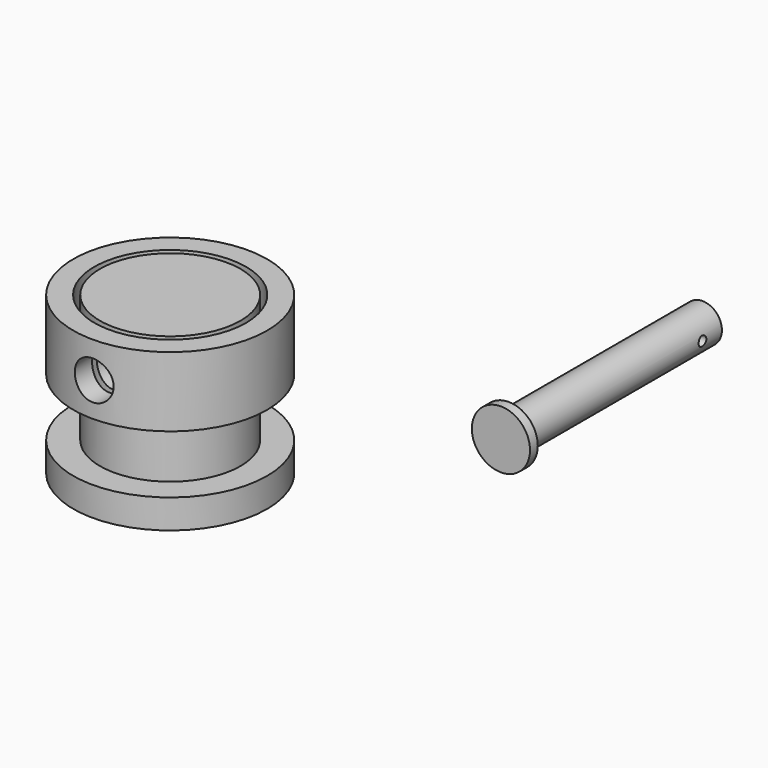
from build123d import *

# Parameters (mm, degrees)
F0_R          = 10
F0_R_2        = 7.83
F1_DEPTH      = 7
F1_DEPTH_BACK = 0.2
F3_R          = 7.25
F4_DEPTH      = 7.2
F4_DEPTH_BACK = 6
F5_START      = 6
F3_R_2        = 10
F3_R_3        = 7.83
F5_DEPTH      = 3
F2_R          = 2
F10_DEPTH     = 93.8892550597
F7_R          = 2
F11_DEPTH     = 25
F7_R_2        = 3
F12_DEPTH     = 1
F13_R         = 0.5
F14_DEPTH     = 25


# Not quite as in the source:
# - a feature of the source that left no trace in its solid (it failed there, or was rolled back) is left out


with BuildPart() as f1:
    # F0 (on Top) → F1 (new body, two sides)
    with BuildSketch(Plane.XY) as f1_sk:
        with Locations((-31.695947051, 83.8882550597)):
            Circle(F0_R)
        with Locations((-31.695947051, 83.8882550597)):
            Circle(F0_R_2, mode=Mode.SUBTRACT)
    extrude(amount=F1_DEPTH)
    extrude(f1_sk.sketch, amount=-F1_DEPTH_BACK)


with BuildPart() as f4:
    # F3 (on face) → F4 (new body, two sides)
    with BuildSketch(Plane(origin=(0, 0, -0.2), x_dir=(1, 0, 0), z_dir=(0, 0, -1))) as f4_sk:
        with Locations((-31.695947051, -83.8882550597)):
            Circle(F3_R)
    extrude(amount=-F4_DEPTH)
    extrude(f4_sk.sketch, amount=F4_DEPTH_BACK)

    # F3 (on face) → F5 (join)
    with BuildSketch(Plane(origin=(0, 0, -0.2), x_dir=(1, 0, 0), z_dir=(0, 0, -1)).offset(F5_START)):
        with Locations((-31.695947051, -83.8882550597)):
            Circle(F3_R_2)
        with Locations((-31.695947051, -83.8882550597)):
            Circle(F3_R_3, mode=Mode.SUBTRACT)
        with Locations((-31.695947051, -83.8882550597)):
            Circle(F3_R_3)
        with Locations((-31.695947051, -83.8882550597)):
            Circle(F3_R, mode=Mode.SUBTRACT)
        with Locations((-31.695947051, -83.8882550597)):
            Circle(F3_R)
    extrude(amount=F5_DEPTH)


with BuildPart() as f10_tool:
    # F2 (on Front) → F10 (new body, through all)
    with BuildSketch(Plane.XZ):
        with Locations((-31.695947051, 3.3)):
            Circle(F2_R)
    extrude(amount=-F10_DEPTH)


with BuildPart() as f1_1:
    add(f1.part)

    # F10: cut by f10_tool
    add(f10_tool.part, mode=Mode.SUBTRACT)


with BuildPart() as f4_1:
    add(f4.part)

    # F10: cut by f10_tool
    add(f10_tool.part, mode=Mode.SUBTRACT)


with BuildPart() as f11:
    # F7 (on offset) → F11 (new body)
    with BuildSketch(Plane.XZ.offset(-70)):
        with Locations((14.3349738792, 14.8918386549)):
            Circle(F7_R)
    extrude(amount=-F11_DEPTH)

    # F7 (on offset) → F12 (join)
    with BuildSketch(Plane.XZ.offset(-70)):
        with Locations((14.3349738792, 14.8918386549)):
            Circle(F7_R_2)
        with Locations((14.3349738792, 14.8918386549)):
            Circle(F7_R, mode=Mode.SUBTRACT)
        with Locations((14.3349738792, 14.8918386549)):
            Circle(F7_R)
    extrude(amount=F12_DEPTH)

    # F13 (on Right) → F14 (cut)
    with BuildSketch(Plane.YZ):
        with Locations((92.5, 14.8918386549)):
            Circle(F13_R)
    extrude(amount=F14_DEPTH, mode=Mode.SUBTRACT)


solid = Compound([f1_1.part, f4_1.part, f11.part])
